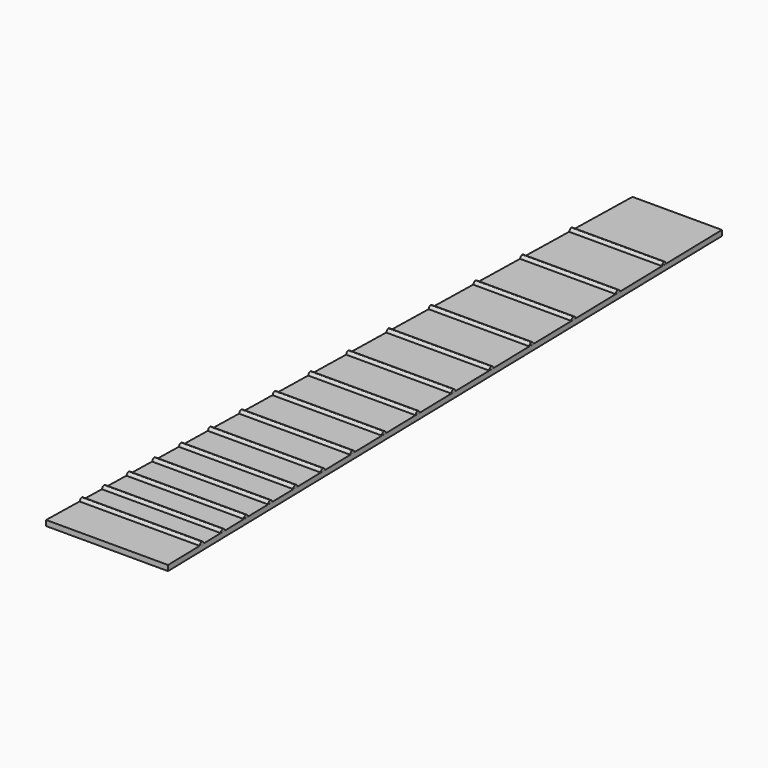
from build123d import *

# Parameters (mm, degrees)
F1_DEPTH     = 2
F2_W         = 44.2697719236
F2_H         = 2
F2_W_2       = 43.7677401211
F2_W_3       = 43.2657083186
F2_W_4       = 42.7408568887
F2_W_5       = 42.1931858314
F2_W_6       = 41.5998755193
F2_W_7       = 40.9609259524
F2_W_8       = 40.2763371308
F2_W_9       = 39.5461090544
F2_W_10      = 38.7702417233
F2_W_11      = 37.9487351373
F2_W_12      = 37.0815892966
F2_W_13      = 36.1688042011
F2_W_14      = 35.2103798508
F2_W_15      = 34.2063162458
F3_DEPTH     = 1
F4_T1_DEPTH  = 50.2158074986
F4_T3_DEPTH  = 3.0186569416
F4_T5_DEPTH  = 47.197150557
F4_T7_DEPTH  = 49.7137756961
F4_T9_DEPTH  = 49.2117438936
F4_T11_DEPTH = 48.6868924637
F4_T13_DEPTH = 48.1392214064
F4_T15_DEPTH = 47.5459110943
F4_T17_DEPTH = 46.9069615275
F4_T19_DEPTH = 46.2223727058
F4_T21_DEPTH = 45.4921446294
F4_T23_DEPTH = 44.7162772983
F4_T25_DEPTH = 43.8947707123
F4_T27_DEPTH = 43.0276248716
F4_T29_DEPTH = 42.1148397761
F4_T31_DEPTH = 41.1564154259
F4_T33_DEPTH = 40.1523518208


# Not quite as in the source:
# - a fillet or chamfer that OpenCascade refuses, or shapes differently, is made with other operations: its cross-section is extruded or revolved along the edge and cut away or added


with BuildPart() as f1:
    # F0 (on Top) → F1 (new body)
    with BuildSketch(Plane.XY):
        Polygon((17.9405650105, 218.366242675), (-15.0594349895, 218.366242675), (-21.0594349895, -44.5653073527), (23.9405650105, -44.5653073527), align=None)
    extrude(amount=F1_DEPTH)

    # F2 (on face) → F3 (join)
    with BuildSketch(Plane.XY.offset(2)):
        with Locations((1.4633846378, -28.5653073527)):
            Rectangle(F2_W, F2_H)
        with Locations((1.4405650105, -18.5653073527)):
            Rectangle(F2_W_2, F2_H)
        with Locations((1.4405650105, -7.5653073527)):
            Rectangle(F2_W_3, F2_H)
        with Locations((1.4405650105, 3.9346926473)):
            Rectangle(F2_W_4, F2_H)
        with Locations((1.4405650105, 15.9346926473)):
            Rectangle(F2_W_5, F2_H)
        with Locations((1.4405650105, 28.9346926473)):
            Rectangle(F2_W_6, F2_H)
        with Locations((1.4405650105, 42.9346926473)):
            Rectangle(F2_W_7, F2_H)
        with Locations((1.4405650105, 57.9346926473)):
            Rectangle(F2_W_8, F2_H)
        with Locations((1.4405650105, 73.9346926473)):
            Rectangle(F2_W_9, F2_H)
        with Locations((1.4405650105, 90.9346926473)):
            Rectangle(F2_W_10, F2_H)
        with Locations((1.4405650105, 108.9346926473)):
            Rectangle(F2_W_11, F2_H)
        with Locations((1.4405650105, 127.9346926473)):
            Rectangle(F2_W_12, F2_H)
        with Locations((1.4405650105, 147.9346926473)):
            Rectangle(F2_W_13, F2_H)
        with Locations((1.4405650105, 168.9346926473)):
            Rectangle(F2_W_14, F2_H)
        with Locations((1.4405650105, 190.9346926473)):
            Rectangle(F2_W_15, F2_H)
    extrude(amount=F3_DEPTH)

    # F4: fillet of radius 1.2071067812 on 30 edges, made by hand

    # F4_s2 → F4_t1 (cut)
    with BuildSketch(Plane.YZ.offset(-23.6445191115)):
        with BuildLine():
            ThreePointArc((-29.5653073527, 2), (-29.1529872247, 2.7167727513), (-28.3761002377, 3))
            Line((-28.3761002377, 3), (-29.5653073527, 3))
            Line((-29.5653073527, 3), (-29.5653073527, 2))
        make_face()
    extrude(amount=F4_T1_DEPTH, mode=Mode.SUBTRACT)

    # F4_s4 → F4_t3 (cut)
    with BuildSketch(Plane.YZ.offset(23.5526314455)):
        with BuildLine():
            ThreePointArc((-27.5653073527, 2), (-27.9776274807, 2.7167727513), (-28.7545144677, 3))
            Line((-28.7545144677, 3), (-27.5653073527, 3))
            Line((-27.5653073527, 3), (-27.5653073527, 2))
        make_face()
    extrude(amount=F4_T3_DEPTH, mode=Mode.SUBTRACT)

    # F4_s6 → F4_t5 (cut)
    with BuildSketch(Plane.YZ.offset(-23.6445191115)):
        with BuildLine():
            ThreePointArc((-27.5653073527, 2), (-27.9776274807, 2.7167727513), (-28.7545144677, 3))
            Line((-28.7545144677, 3), (-27.5653073527, 3))
            Line((-27.5653073527, 3), (-27.5653073527, 2))
        make_face()
    extrude(amount=F4_T5_DEPTH, mode=Mode.SUBTRACT)

    # F4_s8 → F4_t7 (cut)
    with BuildSketch(Plane.YZ.offset(-23.4163228376)):
        with BuildLine():
            ThreePointArc((-19.5653073527, 2), (-19.1529872247, 2.7167727513), (-18.3761002377, 3))
            Line((-18.3761002377, 3), (-19.5653073527, 3))
            Line((-19.5653073527, 3), (-19.5653073527, 2))
        make_face()
        with BuildLine():
            ThreePointArc((-17.5653073527, 2), (-17.9776274807, 2.7167727513), (-18.7545144677, 3))
            Line((-18.7545144677, 3), (-17.5653073527, 3))
            Line((-17.5653073527, 3), (-17.5653073527, 2))
        make_face()
    extrude(amount=F4_T7_DEPTH, mode=Mode.SUBTRACT)

    # F4_s10 → F4_t9 (cut)
    with BuildSketch(Plane.YZ.offset(-23.1653069363)):
        with BuildLine():
            ThreePointArc((-8.5653073527, 2), (-8.1529872247, 2.7167727513), (-7.3761002377, 3))
            Line((-7.3761002377, 3), (-8.5653073527, 3))
            Line((-8.5653073527, 3), (-8.5653073527, 2))
        make_face()
        with BuildLine():
            ThreePointArc((-6.5653073527, 2), (-6.9776274807, 2.7167727513), (-7.7545144677, 3))
            Line((-7.7545144677, 3), (-6.5653073527, 3))
            Line((-6.5653073527, 3), (-6.5653073527, 2))
        make_face()
    extrude(amount=F4_T9_DEPTH, mode=Mode.SUBTRACT)

    # F4_s12 → F4_t11 (cut)
    with BuildSketch(Plane.YZ.offset(-22.9028812214)):
        with BuildLine():
            ThreePointArc((2.9346926473, 2), (3.3470127753, 2.7167727513), (4.1238997623, 3))
            Line((4.1238997623, 3), (2.9346926473, 3))
            Line((2.9346926473, 3), (2.9346926473, 2))
        make_face()
        with BuildLine():
            ThreePointArc((4.9346926473, 2), (4.5223725193, 2.7167727513), (3.7454855323, 3))
            Line((3.7454855323, 3), (4.9346926473, 3))
            Line((4.9346926473, 3), (4.9346926473, 2))
        make_face()
    extrude(amount=F4_T11_DEPTH, mode=Mode.SUBTRACT)

    # F4_s14 → F4_t13 (cut)
    with BuildSketch(Plane.YZ.offset(-22.6290456927)):
        with BuildLine():
            ThreePointArc((14.9346926473, 2), (15.3470127753, 2.7167727513), (16.1238997623, 3))
            Line((16.1238997623, 3), (14.9346926473, 3))
            Line((14.9346926473, 3), (14.9346926473, 2))
        make_face()
        with BuildLine():
            ThreePointArc((16.9346926473, 2), (16.5223725193, 2.7167727513), (15.7454855323, 3))
            Line((15.7454855323, 3), (16.9346926473, 3))
            Line((16.9346926473, 3), (16.9346926473, 2))
        make_face()
    extrude(amount=F4_T13_DEPTH, mode=Mode.SUBTRACT)

    # F4_s16 → F4_t15 (cut)
    with BuildSketch(Plane.YZ.offset(-22.3323905367)):
        with BuildLine():
            ThreePointArc((27.9346926473, 2), (28.3470127753, 2.7167727513), (29.1238997623, 3))
            Line((29.1238997623, 3), (27.9346926473, 3))
            Line((27.9346926473, 3), (27.9346926473, 2))
        make_face()
        with BuildLine():
            ThreePointArc((29.9346926473, 2), (29.5223725193, 2.7167727513), (28.7454855323, 3))
            Line((28.7454855323, 3), (29.9346926473, 3))
            Line((29.9346926473, 3), (29.9346926473, 2))
        make_face()
    extrude(amount=F4_T15_DEPTH, mode=Mode.SUBTRACT)

    # F4_s18 → F4_t17 (cut)
    with BuildSketch(Plane.YZ.offset(-22.0129157533)):
        with BuildLine():
            ThreePointArc((41.9346926473, 2), (42.3470127753, 2.7167727513), (43.1238997623, 3))
            Line((43.1238997623, 3), (41.9346926473, 3))
            Line((41.9346926473, 3), (41.9346926473, 2))
        make_face()
        with BuildLine():
            ThreePointArc((43.9346926473, 2), (43.5223725193, 2.7167727513), (42.7454855323, 3))
            Line((42.7454855323, 3), (43.9346926473, 3))
            Line((43.9346926473, 3), (43.9346926473, 2))
        make_face()
    extrude(amount=F4_T17_DEPTH, mode=Mode.SUBTRACT)

    # F4_s20 → F4_t19 (cut)
    with BuildSketch(Plane.YZ.offset(-21.6706213425)):
        with BuildLine():
            ThreePointArc((56.9346926473, 2), (57.3470127753, 2.7167727513), (58.1238997623, 3))
            Line((58.1238997623, 3), (56.9346926473, 3))
            Line((56.9346926473, 3), (56.9346926473, 2))
        make_face()
        with BuildLine():
            ThreePointArc((58.9346926473, 2), (58.5223725193, 2.7167727513), (57.7454855323, 3))
            Line((57.7454855323, 3), (58.9346926473, 3))
            Line((58.9346926473, 3), (58.9346926473, 2))
        make_face()
    extrude(amount=F4_T19_DEPTH, mode=Mode.SUBTRACT)

    # F4_s22 → F4_t21 (cut)
    with BuildSketch(Plane.YZ.offset(-21.3055073043)):
        with BuildLine():
            ThreePointArc((72.9346926473, 2), (73.3470127753, 2.7167727513), (74.1238997623, 3))
            Line((74.1238997623, 3), (72.9346926473, 3))
            Line((72.9346926473, 3), (72.9346926473, 2))
        make_face()
        with BuildLine():
            ThreePointArc((74.9346926473, 2), (74.5223725193, 2.7167727513), (73.7454855323, 3))
            Line((73.7454855323, 3), (74.9346926473, 3))
            Line((74.9346926473, 3), (74.9346926473, 2))
        make_face()
    extrude(amount=F4_T21_DEPTH, mode=Mode.SUBTRACT)

    # F4_s24 → F4_t23 (cut)
    with BuildSketch(Plane.YZ.offset(-20.9175736387)):
        with BuildLine():
            ThreePointArc((89.9346926473, 2), (90.3470127753, 2.7167727513), (91.1238997623, 3))
            Line((91.1238997623, 3), (89.9346926473, 3))
            Line((89.9346926473, 3), (89.9346926473, 2))
        make_face()
        with BuildLine():
            ThreePointArc((91.9346926473, 2), (91.5223725193, 2.7167727513), (90.7454855323, 3))
            Line((90.7454855323, 3), (91.9346926473, 3))
            Line((91.9346926473, 3), (91.9346926473, 2))
        make_face()
    extrude(amount=F4_T23_DEPTH, mode=Mode.SUBTRACT)

    # F4_s26 → F4_t25 (cut)
    with BuildSketch(Plane.YZ.offset(-20.5068203457)):
        with BuildLine():
            ThreePointArc((107.9346926473, 2), (108.3470127753, 2.7167727513), (109.1238997623, 3))
            Line((109.1238997623, 3), (107.9346926473, 3))
            Line((107.9346926473, 3), (107.9346926473, 2))
        make_face()
        with BuildLine():
            ThreePointArc((109.9346926473, 2), (109.5223725193, 2.7167727513), (108.7454855323, 3))
            Line((108.7454855323, 3), (109.9346926473, 3))
            Line((109.9346926473, 3), (109.9346926473, 2))
        make_face()
    extrude(amount=F4_T25_DEPTH, mode=Mode.SUBTRACT)

    # F4_s28 → F4_t27 (cut)
    with BuildSketch(Plane.YZ.offset(-20.0732474254)):
        with BuildLine():
            ThreePointArc((126.9346926473, 2), (127.3470127753, 2.7167727513), (128.1238997623, 3))
            Line((128.1238997623, 3), (126.9346926473, 3))
            Line((126.9346926473, 3), (126.9346926473, 2))
        make_face()
        with BuildLine():
            ThreePointArc((128.9346926473, 2), (128.5223725193, 2.7167727513), (127.7454855323, 3))
            Line((127.7454855323, 3), (128.9346926473, 3))
            Line((128.9346926473, 3), (128.9346926473, 2))
        make_face()
    extrude(amount=F4_T27_DEPTH, mode=Mode.SUBTRACT)

    # F4_s30 → F4_t29 (cut)
    with BuildSketch(Plane.YZ.offset(-19.6168548776)):
        with BuildLine():
            ThreePointArc((146.9346926473, 2), (147.3470127753, 2.7167727513), (148.1238997623, 3))
            Line((148.1238997623, 3), (146.9346926473, 3))
            Line((146.9346926473, 3), (146.9346926473, 2))
        make_face()
        with BuildLine():
            ThreePointArc((148.9346926473, 2), (148.5223725193, 2.7167727513), (147.7454855323, 3))
            Line((147.7454855323, 3), (148.9346926473, 3))
            Line((148.9346926473, 3), (148.9346926473, 2))
        make_face()
    extrude(amount=F4_T29_DEPTH, mode=Mode.SUBTRACT)

    # F4_s32 → F4_t31 (cut)
    with BuildSketch(Plane.YZ.offset(-19.1376427025)):
        with BuildLine():
            ThreePointArc((167.9346926473, 2), (168.3470127753, 2.7167727513), (169.1238997623, 3))
            Line((169.1238997623, 3), (167.9346926473, 3))
            Line((167.9346926473, 3), (167.9346926473, 2))
        make_face()
        with BuildLine():
            ThreePointArc((169.9346926473, 2), (169.5223725193, 2.7167727513), (168.7454855323, 3))
            Line((168.7454855323, 3), (169.9346926473, 3))
            Line((169.9346926473, 3), (169.9346926473, 2))
        make_face()
    extrude(amount=F4_T31_DEPTH, mode=Mode.SUBTRACT)

    # F4_s34 → F4_t33 (cut)
    with BuildSketch(Plane.YZ.offset(-18.6356109)):
        with BuildLine():
            ThreePointArc((189.9346926473, 2), (190.3470127753, 2.7167727513), (191.1238997623, 3))
            Line((191.1238997623, 3), (189.9346926473, 3))
            Line((189.9346926473, 3), (189.9346926473, 2))
        make_face()
        with BuildLine():
            ThreePointArc((191.9346926473, 2), (191.5223725193, 2.7167727513), (190.7454855323, 3))
            Line((190.7454855323, 3), (191.9346926473, 3))
            Line((191.9346926473, 3), (191.9346926473, 2))
        make_face()
    extrude(amount=F4_T33_DEPTH, mode=Mode.SUBTRACT)


solid = f1.part
